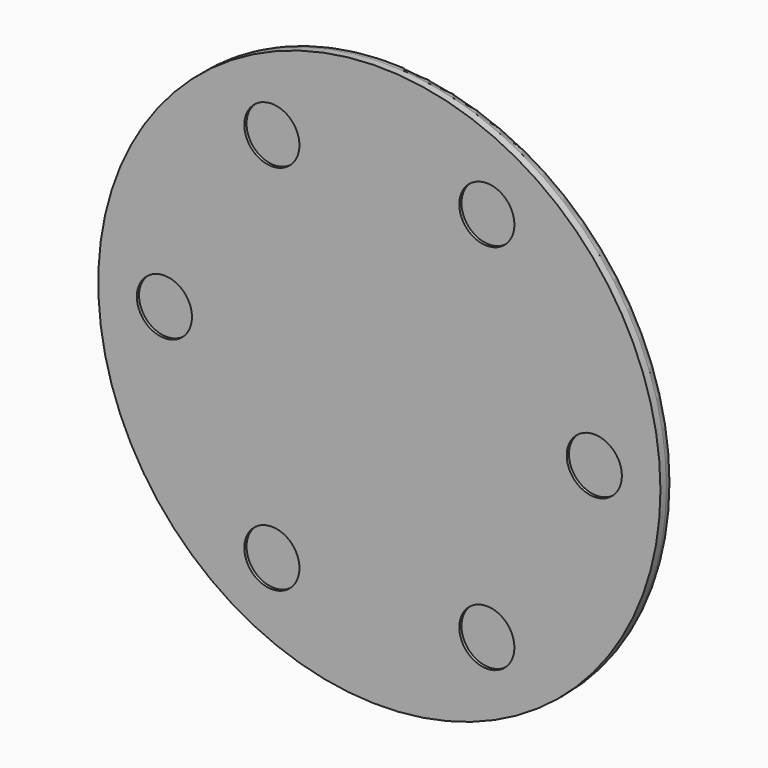
from build123d import *

# Parameters (mm, degrees)
F2_R            = 5
F3_DEPTH        = 0.5
F3_COPIES_COUNT = 6


# Not quite as in the source:
# - a pattern or mirror of a feature is missing from the dataset's text; its kind, count and spacing are read off the source's solid


with BuildPart() as f1:
    # F0 (on Top) → F1 (revolve)
    with BuildSketch(Plane.XY):
        with BuildLine():
            Line((0, 6), (0, 0))
            Line((0, 0), (51, 0))
            Line((51, 0), (51, 1.3443025184))
            ThreePointArc((51, 1.3443025184), (50.5372887774, 2.6236551731), (49.363256785, 3.3110369967))
            ThreePointArc((49.363256785, 3.3110369967), (34.7430608343, 5.3263557546), (20, 6))
            Line((20, 6), (0, 6))
        make_face()
    revolve(axis=Axis((0, 3, 0), (0, 1, 0)))

    # F2 (on face) → F3 (cut)
    with BuildSketch(Plane.XZ):
        with Locations((39, 0)):
            Circle(F2_R)
    f3 = extrude(amount=-F3_DEPTH, mode=Mode.SUBTRACT)

    # F3_copies: F3 ×6 about axis
    f3_copies_axis = Axis((0, 0, 0), (0, 1, 0))
    for i in range(1, F3_COPIES_COUNT):
        add(f3.rotate(f3_copies_axis, i * 360 / F3_COPIES_COUNT), mode=Mode.SUBTRACT)


solid = f1.part
